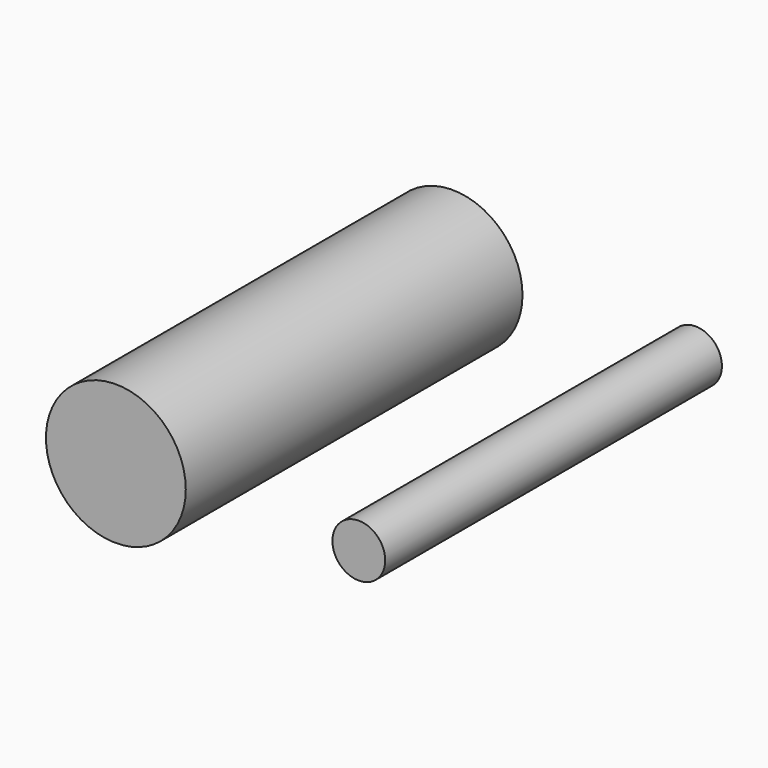
from build123d import *

# Parameters (mm, degrees)
F4_R     = 4.983561163
F5_DEPTH = 30
F6_R     = 1.882044971
F7_DEPTH = 30


# Not quite as in the source:
# - the program builds the solid bodies; features that only make, move or delete a surface that nothing else refers to are left out


with BuildPart() as f5:
    # F4 (on Front) → F5 (new body)
    with BuildSketch(Plane.XZ):
        with Locations((-8.6584175006, 65.3990134597)):
            Circle(F4_R)
    extrude(amount=F5_DEPTH)


with BuildPart() as f7:
    # F6 (on Front) → F7 (new body)
    with BuildSketch(Plane.XZ):
        with Locations((8.6574237794, 65.5710920691)):
            Circle(F6_R)
    extrude(amount=F7_DEPTH)


solid = Compound([f5.part, f7.part])
